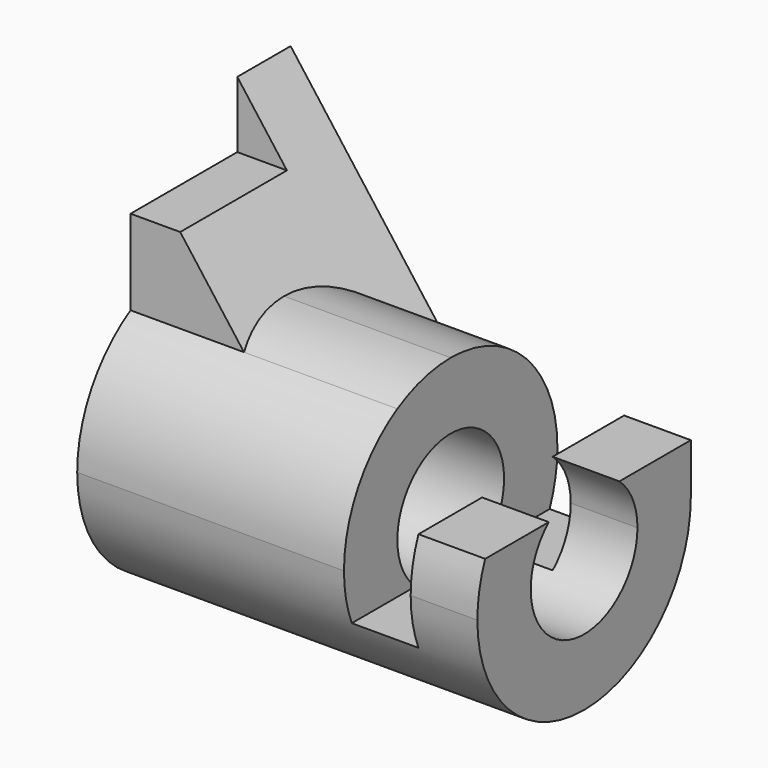
from build123d import *

# Parameters (mm, degrees)
F0_W         = 76.2
F0_H         = 76.2
F1_DEPTH     = 50.8
F2_R         = 12.7
F3_DEPTH     = 76.201
F5_DEPTH     = 25.4
F6_DEPTH     = 50.801
F7_R         = 25.39999
F9_DEPTH     = 25.4
F10_DEPTH    = 76.201
F11_T1_DEPTH = 203.2


# Not quite as in the source:
# - a fillet or chamfer that OpenCascade refuses, or shapes differently, is made with other operations: its cross-section is extruded or revolved along the edge and cut away or added
# - a fillet or chamfer is up to 0.001 mm smaller than in the source, because OpenCascade refuses the exact size


with BuildPart() as f1:
    # F0 (on Front) → F1 (new body)
    with BuildSketch(Plane.XZ):
        with Locations((38.1, 38.1)):
            Rectangle(F0_W, F0_H)
    extrude(amount=F1_DEPTH)

    # F2 (on face) → F3 (cut, through all)
    with BuildSketch(Plane.YZ.offset(76.2)):
        with Locations((-25.4, 25.4)):
            Circle(F2_R)
    extrude(amount=-F3_DEPTH, mode=Mode.SUBTRACT)

    # F4 (on face) → F5 (cut)
    with BuildSketch(Plane.XZ.offset(50.8)):
        Polygon((63.5, 34.925), (76.2, 34.925), (76.2, 76.2), (0, 76.2), (19.05, 50.8), (50.8, 50.8), (50.8, 15.875), (63.5, 15.875), align=None)
    extrude(amount=-F5_DEPTH, mode=Mode.SUBTRACT)

    # F4 (on face) → F6 (cut, through all)
    with BuildSketch(Plane.XZ.offset(50.8)):
        Polygon((63.5, 34.925), (76.2, 34.925), (76.2, 76.2), (0, 76.2), (19.05, 50.8), (50.8, 50.8), (50.8, 15.875), (63.5, 15.875), align=None)
    extrude(amount=-F6_DEPTH, mode=Mode.SUBTRACT)

    # F7 (radius 25.4 in the source; OpenCascade refuses exactly that, so slightly less here)
    f7_edges = [f1.edges().sort_by_distance(p)[0] for p in [
        (34.925, -50.8, 50.8),
        (34.925, 0, 50.8),
    ]]
    fillet(f7_edges, radius=F7_R)

    # F8 (on face) → F9 (cut)
    with BuildSketch(Plane(origin=(0, 0, 0), x_dir=(0, -1, 0), z_dir=(-1, 0, 0))):
        with BuildLine():
            Line((50.8, 76.2), (12.7, 76.2))
            Line((12.7, 76.2), (12.7, 63.5934035911))
            Line((12.7, 63.5934035911), (38.1, 63.5934035911))
            Line((38.1, 63.5934035911), (38.1, 47.3970452561))
            ThreePointArc((38.1, 47.3970452561), (47.3970452561, 38.1), (50.8, 25.4))
            Line((50.8, 25.4), (50.8, 76.2))
        make_face()
    extrude(amount=-F9_DEPTH, mode=Mode.SUBTRACT)

    # F8 (on face) → F10 (cut, through all)
    with BuildSketch(Plane(origin=(0, 0, 0), x_dir=(0, -1, 0), z_dir=(-1, 0, 0))):
        with BuildLine():
            Line((50.8, 76.2), (12.7, 76.2))
            Line((12.7, 76.2), (12.7, 63.5934035911))
            Line((12.7, 63.5934035911), (38.1, 63.5934035911))
            Line((38.1, 63.5934035911), (38.1, 47.3970452561))
            ThreePointArc((38.1, 47.3970452561), (47.3970452561, 38.1), (50.8, 25.4))
            Line((50.8, 25.4), (50.8, 76.2))
        make_face()
    extrude(amount=-F10_DEPTH, mode=Mode.SUBTRACT)

    # F11: fillet of radius 25.4 on 2 edges, made by hand

    # F11_s2 → F11_t1 (cut)
    with BuildSketch(Plane.YZ.offset(-63.5)):
        with BuildLine():
            ThreePointArc((-50.8, 25.4), (-43.3605122421, 7.4394877579), (-25.4, 0))
            Line((-25.4, 0), (-50.8, 0))
            Line((-50.8, 0), (-50.8, 25.4))
        make_face()
        with BuildLine():
            ThreePointArc((0, 25.4), (-7.4394877579, 7.4394877579), (-25.4, 0))
            Line((-25.4, 0), (0, 0))
            Line((0, 0), (0, 25.4))
        make_face()
    extrude(amount=F11_T1_DEPTH, mode=Mode.SUBTRACT)


solid = f1.part
